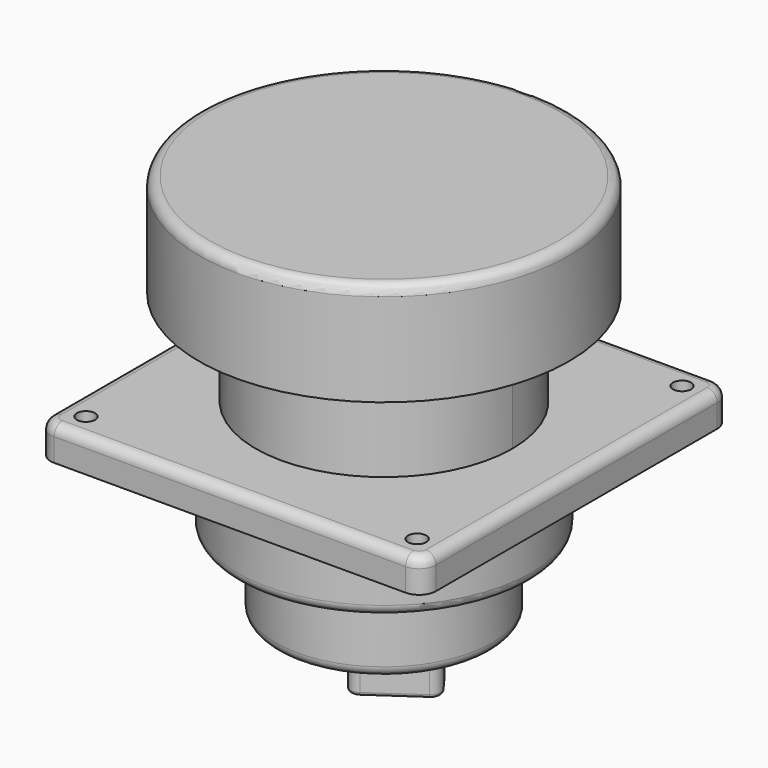
from build123d import *

# Parameters (mm, degrees)
F0_R         = 2.7
F1_DEPTH     = 9.8
F0_W         = 34
F0_H         = 4
F2_DEPTH     = 38
F3_R         = 54.75
F4_DEPTH     = 30.5
F5_R         = 3
F5_2_R       = 3
F6_T1_DEPTH  = 22.3
F6_T3_DEPTH  = 59
F6_T6_ANGLE  = 90
F6_T8_ANGLE  = 90
F6_T10_ANGLE = 90
F6_T12_ANGLE = 90
F8_DEPTH     = 74.001
F9_T1_DEPTH  = 70.646815
F10_R        = 43.55
F11_DEPTH    = 23.75
F12_R        = 32
F13_DEPTH    = 22
F15_DEPTH    = 13.25
F16_DEPTH    = 10.4
F17_R        = 3
F18_R        = 1


# Not quite as in the source:
# - a fillet or chamfer that OpenCascade refuses, or shapes differently, is made with other operations: its cross-section is extruded or revolved along the edge and cut away or added


with BuildPart() as f1:
    # F0 (on Top) → F1 (new body)
    with BuildSketch(Plane.XY):
        with BuildLine():
            Line((-57, -57), (57, -57))
            Line((57, -57), (57, 57))
            Line((57, 57), (17, 57))
            Line((17, 57), (17, 41))
            Line((17, 41), (17, 33.985291))
            ThreePointArc((17, 33.985291), (32.32646, 19.974984), (38, 0))
            ThreePointArc((38, 0), (-19.974984, -32.32646), (-17, 33.985291))
            Line((-17, 33.985291), (-17, 41))
            Line((-17, 41), (-17, 57))
            Line((-17, 57), (-57, 57))
            Line((-57, 57), (-57, -57))
        make_face()
        with Locations((-49, -49)):
            Circle(F0_R, mode=Mode.SUBTRACT)
        with Locations((49, -49)):
            Circle(F0_R, mode=Mode.SUBTRACT)
        with Locations((-49, 49)):
            Circle(F0_R, mode=Mode.SUBTRACT)
        with Locations((49, 49)):
            Circle(F0_R, mode=Mode.SUBTRACT)
    extrude(amount=F1_DEPTH)

    # F0 (on Top) → F2 (join)
    with BuildSketch(Plane.XY):
        with Locations((0, 59)):
            Rectangle(F0_W, F0_H)
        with BuildLine():
            Line((17, 41), (17, 57))
            Line((17, 57), (-17, 57))
            Line((-17, 57), (-17, 41))
            Line((-17, 41), (-17, 33.985291))
            ThreePointArc((-17, 33.985291), (0, 38), (17, 33.985291))
            Line((17, 33.985291), (17, 41))
        make_face()
        with BuildLine():
            ThreePointArc((38, 0), (32.32646, 19.974984), (17, 33.985291))
            ThreePointArc((17, 33.985291), (0, 38), (-17, 33.985291))
            ThreePointArc((-17, 33.985291), (-19.974984, -32.32646), (38, 0))
        make_face()
    extrude(amount=F2_DEPTH)

    # F5
    f5_edges = [f1.edges().sort_by_distance(p)[0] for p in [
        (-57, 0, 9.8),
        (0, -57, 9.8),
        (57, 0, 9.8),
        (37, 57, 9.8),
        (-37, 57, 9.8),
    ]]
    fillet(f5_edges, radius=F5_R)

    # F6: fillet of radius 5 on 5 edges, made by hand

    # F6_s2 → F6_t1 (cut)
    with BuildSketch(Plane.XY.offset(-12.5)):
        with BuildLine():
            ThreePointArc((57, 52), (55.535534, 55.535534), (52, 57))
            Line((52, 57), (57, 57))
            Line((57, 57), (57, 52))
        make_face()
        with BuildLine():
            ThreePointArc((-57, 52), (-55.535534, 55.535534), (-52, 57))
            Line((-52, 57), (-57, 57))
            Line((-57, 57), (-57, 52))
        make_face()
        with BuildLine():
            ThreePointArc((52, -57), (55.535534, -55.535534), (57, -52))
            Line((57, -52), (57, -57))
            Line((57, -57), (52, -57))
        make_face()
        with BuildLine():
            ThreePointArc((-52, -57), (-55.535534, -55.535534), (-57, -52))
            Line((-57, -52), (-57, -57))
            Line((-57, -57), (-52, -57))
        make_face()
    extrude(amount=F6_T1_DEPTH, mode=Mode.SUBTRACT)

    # F6_s4 → F6_t3 (cut)
    with BuildSketch(Plane.YZ.offset(-29.5)):
        with BuildLine():
            ThreePointArc((61, 33), (59.535534, 36.535534), (56, 38))
            Line((56, 38), (61, 38))
            Line((61, 38), (61, 33))
        make_face()
    extrude(amount=F6_T3_DEPTH, mode=Mode.SUBTRACT)

    # F6_s5 → F6_t6 (revolve, cut)
    with BuildSketch(Plane.XZ.offset(52)):
        with BuildLine():
            ThreePointArc((-54, 9.8), (-56.12132, 8.92132), (-57, 6.8))
            Line((-57, 6.8), (-57, 9.8))
            Line((-57, 9.8), (-54, 9.8))
        make_face()
    revolve(axis=Axis((-52, -52, 9.8), (0, 0, 1)), revolution_arc=F6_T6_ANGLE, mode=Mode.SUBTRACT)

    # F6_s7 → F6_t8 (revolve, cut)
    with BuildSketch(Plane.YZ.offset(52)):
        with BuildLine():
            ThreePointArc((-54, 9.8), (-56.12132, 8.92132), (-57, 6.8))
            Line((-57, 6.8), (-57, 9.8))
            Line((-57, 9.8), (-54, 9.8))
        make_face()
    revolve(axis=Axis((52, -52, 9.8), (0, 0, 1)), revolution_arc=F6_T8_ANGLE, mode=Mode.SUBTRACT)

    # F6_s9 → F6_t10 (revolve, cut)
    with BuildSketch(Plane.YZ.offset(-52)):
        with BuildLine():
            ThreePointArc((54, 9.8), (56.12132, 8.92132), (57, 6.8))
            Line((57, 6.8), (57, 9.8))
            Line((57, 9.8), (54, 9.8))
        make_face()
    revolve(axis=Axis((-52, 52, 9.8), (0, 0, 1)), revolution_arc=F6_T10_ANGLE, mode=Mode.SUBTRACT)

    # F6_s11 → F6_t12 (revolve, cut)
    with BuildSketch(Plane.XZ.offset(-52)):
        with BuildLine():
            ThreePointArc((54, 9.8), (56.12132, 8.92132), (57, 6.8))
            Line((57, 6.8), (57, 9.8))
            Line((57, 9.8), (54, 9.8))
        make_face()
    revolve(axis=Axis((52, 52, 9.8), (0, 0, 1)), revolution_arc=F6_T12_ANGLE, mode=Mode.SUBTRACT)

    # F7 (on face) → F8 (cut, through all)
    with BuildSketch(Plane(origin=(-17, 0, 0), x_dir=(0, -1, 0), z_dir=(-1, 0, 0))):
        with BuildLine():
            Line((-52.05122, 9.8), (-61, 33))
            Line((-61, 33), (-61, 0))
            Line((-61, 0), (-57, 0))
            Line((-57, 0), (-57, 6.8))
            ThreePointArc((-57, 6.8), (-56.12132, 8.92132), (-54, 9.8))
            Line((-54, 9.8), (-52.05122, 9.8))
        make_face()
    extrude(amount=-F8_DEPTH, mode=Mode.SUBTRACT)

    # F9: fillet of radius 5 on 1 edges, made by hand

    # F9_s2 → F9_t1 (cut)
    with BuildSketch(Plane.YZ.offset(-35.323407)):
        with BuildLine():
            ThreePointArc((55.640937, 38), (59.763859, 35.828694), (60.305931, 31.200603))
            Line((60.305931, 31.200603), (60.77243, 31.020663))
            Line((60.77243, 31.020663), (61.466499, 32.82006))
            Line((61.466499, 32.82006), (61.5, 33))
            ThreePointArc((61.5, 33), (56, 38.5), (55.640937, 38.5))
            Line((55.640937, 38.5), (55.640937, 38))
        make_face()
    extrude(amount=F9_T1_DEPTH, mode=Mode.SUBTRACT)

    # F10 (on face) → F11 (join)
    with BuildSketch(Plane.XY):
        Circle(F10_R)
    extrude(amount=-F11_DEPTH)

    # F12 (on face) → F13 (join)
    with BuildSketch(Plane(origin=(0, 0, -23.75), x_dir=(1, 0, 0), z_dir=(0, 0, -1))):
        Circle(F12_R)
    extrude(amount=F13_DEPTH)

    # F14 (on face) → F15 (join)
    with BuildSketch(Plane(origin=(0, 0, -45.75), x_dir=(1, 0, 0), z_dir=(0, 0, -1))):
        Polygon((-6.043476, 1.320423), (3.199485, -14.524652), (10.717843, -10.291299), (1.408572, 5.667451), align=None)
    extrude(amount=F15_DEPTH)

    # F14 (on face) → F16 (join)
    with BuildSketch(Plane(origin=(0, 0, -45.75), x_dir=(1, 0, 0), z_dir=(0, 0, -1))):
        Polygon((0, 12.493231), (18.028848, 0), (24.565879, 8.877769), (6.276854, 21.551292), align=None)
    extrude(amount=F16_DEPTH)

    # F17
    f17_edges = [f1.edges().sort_by_distance(p)[0] for p in [
        (43.55, 0, -11.875),
        (-43.55, 0, 0),
        (-43.55, 0, -23.75),
        (-32, 0, -45.75),
        (24.565879, -8.877769, -50.95),
        (6.276854, -21.551292, -50.95),
        (1.408572, -5.667451, -52.375),
        (10.717843, 10.291299, -52.375),
        (0, -12.493231, -50.95),
        (18.028848, 0, -50.95),
        (-6.043476, -1.320423, -52.375),
        (3.199485, 14.524652, -52.375),
    ]]
    fillet(f17_edges, radius=F17_R)

    # F18
    f18_edges = [f1.edges().sort_by_distance(p)[0] for p in [
        (9.049329, -6.222428, -56.15),
        (1.222694, -12.714984, -56.15),
        (17.834469, -1.166937, -56.15),
        (3.138427, -17.022262, -56.15),
        (21.24627, -4.369496, -56.15),
        (6.498607, -20.328597, -56.15),
        (23.278723, -8.663365, -56.15),
        (15.385445, -15.239422, -56.15),
        (6.05159, 2.292009, -59),
        (9.486975, 9.957328, -59),
        (1.092328, -4.465725, -59),
        (6.918788, 12.430428, -59),
        (-2.317452, -3.493937, -59),
        (3.516507, 13.356246, -59),
        (-4.841749, -1.004179, -59),
        (-1.410554, 6.621728, -59),
    ]]
    fillet(f18_edges, radius=F18_R)


with BuildPart() as f4:
    # F3 (on face) → F4 (new body)
    with BuildSketch(Plane.XY.offset(38)):
        Circle(F3_R)
    extrude(amount=F4_DEPTH)

    # F5#2
    f5_2_edges = [f4.edges().sort_by_distance(p)[0] for p in [
        (-54.75, 0, 68.5),
    ]]
    fillet(f5_2_edges, radius=F5_2_R)


solid = Compound([f1.part, f4.part])
